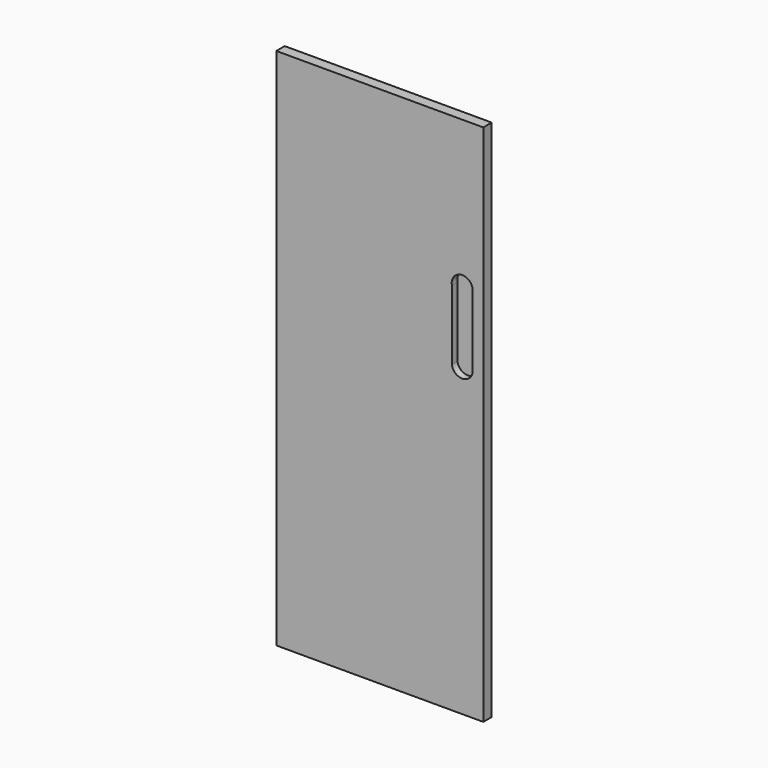
from build123d import *

# Parameters (mm, degrees)
F0_W     = 295
F0_H     = 746
F1_DEPTH = 15
F3_DEPTH = 10


with BuildPart() as f1:
    # F0 (on Front) → F1 (new body)
    with BuildSketch(Plane.XZ):
        Rectangle(F0_W, F0_H)
    extrude(amount=F1_DEPTH)

    # F2 (on face) → F3 (cut)
    with BuildSketch(Plane.XZ.offset(15)):
        with BuildLine():
            ThreePointArc((132.4401133717, 161.6609658553), (132.4850208638, 162.3298136735), (132.5, 163))
            ThreePointArc((132.5, 163), (116.3496874374, 177.9558276604), (102.6764291989, 160.7061498078))
            ThreePointArc((102.6764291989, 160.7061498078), (117.9809511033, 148.0077124482), (132.4401133717, 161.6609658553))
        make_face()
        with BuildLine():
            ThreePointArc((132.4401133717, 161.6609658553), (117.9809511033, 148.0077124482), (102.6764291989, 160.7061498078))
            Line((102.6764291989, 160.7061498078), (102.6764291989, 65.2938501922))
            ThreePointArc((102.6764291989, 65.2938501922), (117.9809511033, 77.9922875518), (132.4401133717, 64.3390341447))
            Line((132.4401133717, 64.3390341447), (132.4401133717, 161.6609658553))
        make_face()
        with BuildLine():
            ThreePointArc((132.4401133717, 64.3390341447), (117.9809511033, 77.9922875518), (102.6764291989, 65.2938501922))
            Line((102.6764291989, 65.2938501922), (102.6764291989, 60.7061498078))
            ThreePointArc((102.6764291989, 60.7061498078), (117.9809511033, 48.0077124482), (132.4401133717, 61.6609658553))
            Line((132.4401133717, 61.6609658553), (132.4401133717, 64.3390341447))
        make_face()
    extrude(amount=-F3_DEPTH, mode=Mode.SUBTRACT)


solid = f1.part
